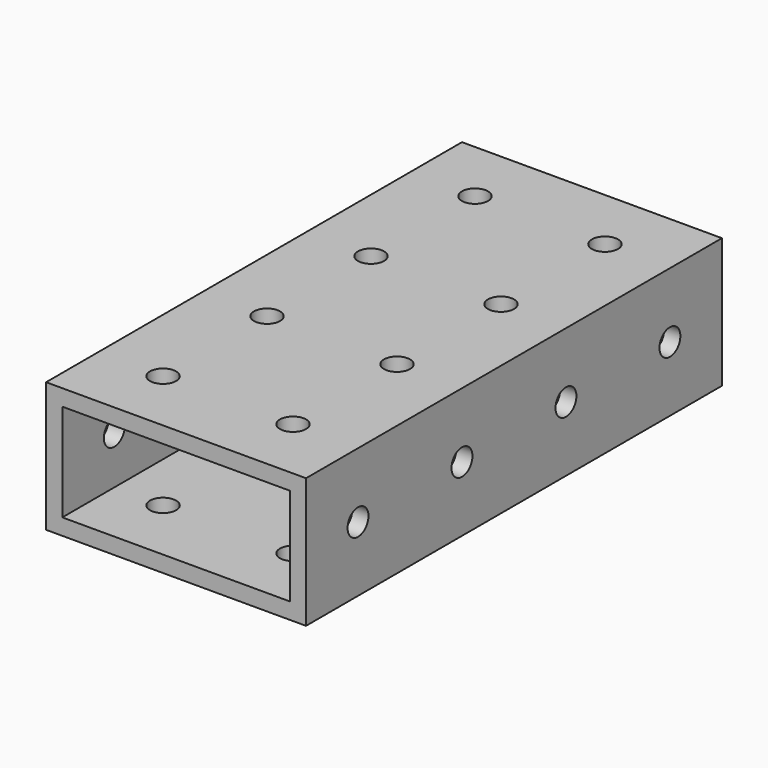
from build123d import *

# Parameters (mm, degrees)
F0_W     = 50.8
F0_H     = 25.4
F0_W_2   = 44.45
F0_H_2   = 19.05
F1_DEPTH = 101.6
F3_D     = 5.1054
F5_D     = 5.1054


# Not quite as in the source:
# - a feature names something its author has since deleted; it is built from what else it names


with BuildPart() as f1:
    # F0 (on Front) → F1 (new body)
    with BuildSketch(Plane.XZ):
        Rectangle(F0_W, F0_H)
        Rectangle(F0_W_2, F0_H_2, mode=Mode.SUBTRACT)
    extrude(amount=F1_DEPTH)

    # F3 (through all)
    with Locations(Plane.XY.offset(12.7)):
        with Locations((-12.7, -88.9), (-12.7, -12.7), (-12.7, -38.1), (-12.7, -63.5), (12.7, -12.7), (12.7, -88.9), (12.7, -38.1), (12.7, -63.5)):
            Hole(F3_D / 2)

    # F5 (through all)
    with Locations(Plane.YZ.offset(25.4)):
        with Locations((-88.9, 0), (-63.5, 0), (-38.1, 0), (-12.7, 0)):
            Hole(F5_D / 2)


solid = f1.part
